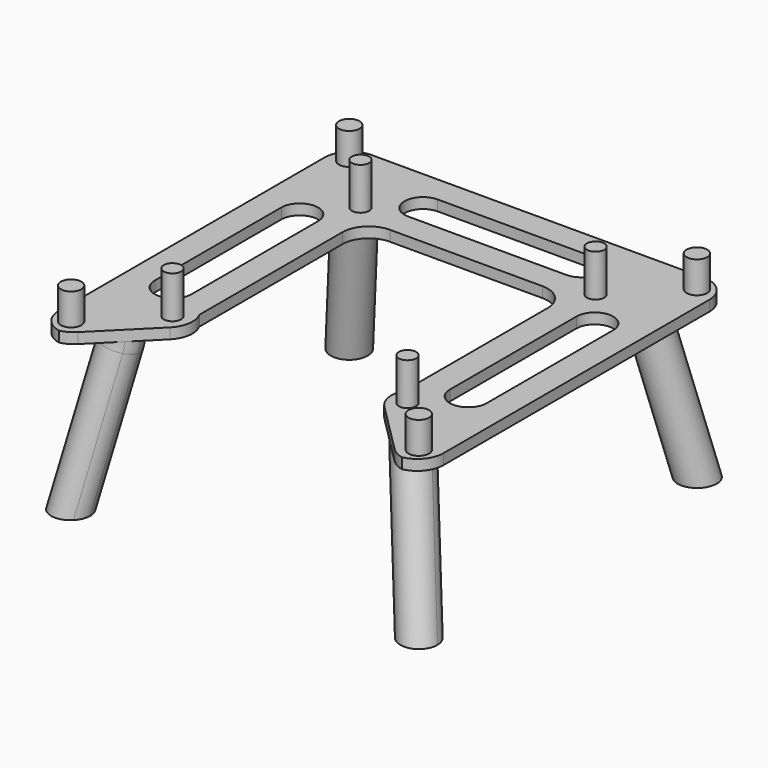
from build123d import *

# Parameters (mm, degrees)
F0_R           = 1.95
F0_R_2         = 1.65
F0_R_3         = 3.5355339059
F1_DEPTH       = 2
F2_T1_DEPTH    = 43.5812984693
F2_T3_DEPTH    = 12.3553390593
F2_T5_DEPTH    = 27
F2_T7_DEPTH    = 2
F3_ANGLE       = 15
F4_DEPTH       = 30
F5_ANGLE       = 15
F6_ANGLE       = 15
F7_ANGLE       = 15
F8_DEPTH       = 30
F9_DEPTH       = 30
F10_DEPTH      = 30
F11_W          = 91.7069762945
F11_H          = 4.37906757
F12_DEPTH      = 40
F12_DEPTH_BACK = 40
F13_DEPTH      = 10
F14_DEPTH      = 8


# Not quite as in the source:
# - a fillet or chamfer that OpenCascade refuses, or shapes differently, is made with other operations: its cross-section is extruded or revolved along the edge and cut away or added


with BuildPart() as f1:
    # F0 (on Top) → F1 (new body)
    with BuildSketch(Plane.XY):
        Polygon((-19.4715728753, 19.4715728753), (19.4715728753, 19.4715728753), (19.4715728753, -19.4715728753), (14.4715728753, -19.4715728753), (25.1386562498, -30.1386562498), (31.5128463018, -36.5128463018), (36.5128463018, -36.5128463018), (36.5128463018, 36.5128463018), (-36.5128463018, 36.5128463018), (-36.5128463018, -36.5128463018), (-31.5128463018, -36.5128463018), (-25.138656198, -30.138656198), (-14.4715728753, -19.4715728753), (-19.4715728753, -19.4715728753), align=None)
        with Locations((-32.9773123959, -32.9773123959)):
            Circle(F0_R, mode=Mode.SUBTRACT)
        with BuildLine():
            ThreePointArc((-24.103122292, -27.638656198), (-24.3722487858, -28.9916464483), (-25.138656198, -30.138656198))
            ThreePointArc((-25.138656198, -30.138656198), (-30.9050636101, -26.2856659476), (-24.103122292, -27.638656198))
        make_face(mode=Mode.SUBTRACT)
        with Locations((-22.3, -22.3)):
            Circle(F0_R_2, mode=Mode.SUBTRACT)
        with Locations((32.9773123959, -32.9773123959)):
            Circle(F0_R, mode=Mode.SUBTRACT)
        with BuildLine():
            ThreePointArc((31.1741901039, -27.638656198), (28.9916464822, -30.9050635961), (25.1386562498, -30.1386562498))
            ThreePointArc((25.1386562498, -30.1386562498), (26.2856659138, -24.3722487998), (31.1741901039, -27.638656198))
        make_face(mode=Mode.SUBTRACT)
        with Locations((22.3, -22.3)):
            Circle(F0_R_2, mode=Mode.SUBTRACT)
        with BuildLine():
            Line((-31.4922095886, -15), (-31.4922095886, 15))
            ThreePointArc((-31.4922095886, 15), (-27.9922095886, 18.5), (-24.4922095886, 15))
            Line((-24.4922095886, 15), (-24.4922095886, -15))
            ThreePointArc((-24.4922095886, -15), (-27.9922095886, -18.5), (-31.4922095886, -15))
        make_face(mode=Mode.SUBTRACT)
        with Locations((-22.3, 22.3)):
            Circle(F0_R_2, mode=Mode.SUBTRACT)
        with Locations((-27.638656198, 27.638656198)):
            Circle(F0_R_3, mode=Mode.SUBTRACT)
        with Locations((-32.9773123959, 32.9773123959)):
            Circle(F0_R, mode=Mode.SUBTRACT)
        with BuildLine():
            Line((31.4922095886, 15), (31.4922095886, -15))
            ThreePointArc((31.4922095886, -15), (27.9922095886, -18.5), (24.4922095886, -15))
            Line((24.4922095886, -15), (24.4922095886, 15))
            ThreePointArc((24.4922095886, 15), (27.9922095886, 18.5), (31.4922095886, 15))
        make_face(mode=Mode.SUBTRACT)
        with BuildLine():
            Line((-15, 31.4922095886), (15, 31.4922095886))
            ThreePointArc((15, 31.4922095886), (18.5, 27.9922095886), (15, 24.4922095886))
            Line((15, 24.4922095886), (-15, 24.4922095886))
            ThreePointArc((-15, 24.4922095886), (-18.5, 27.9922095886), (-15, 31.4922095886))
        make_face(mode=Mode.SUBTRACT)
        with Locations((22.3, 22.3)):
            Circle(F0_R_2, mode=Mode.SUBTRACT)
        with Locations((27.638656198, 27.638656198)):
            Circle(F0_R_3, mode=Mode.SUBTRACT)
        with Locations((32.9773123959, 32.9773123959)):
            Circle(F0_R, mode=Mode.SUBTRACT)
        with BuildLine():
            ThreePointArc((-24.103122292, -27.638656198), (-30.9050636101, -26.2856659476), (-25.138656198, -30.138656198))
            ThreePointArc((-25.138656198, -30.138656198), (-24.3722487858, -28.9916464483), (-24.103122292, -27.638656198))
        make_face()
        with Locations((-27.638656198, 27.638656198)):
            Circle(F0_R_3)
        with BuildLine():
            ThreePointArc((31.1741901039, -27.638656198), (26.2856659138, -24.3722487998), (25.1386562498, -30.1386562498))
            ThreePointArc((25.1386562498, -30.1386562498), (28.9916464822, -30.9050635961), (31.1741901039, -27.638656198))
        make_face()
        with Locations((27.638656198, 27.638656198)):
            Circle(F0_R_3)
    extrude(amount=F1_DEPTH)

    # F2: fillet of radius 5 on 10 edges, made by hand

    # F2_s2 → F2_t1 (cut)
    with BuildSketch(Plane.XY.offset(-20.7906492346)):
        with BuildLine():
            ThreePointArc((-20.3520564989, -25.3520564989), (-18.9427128058, -22.5569181158), (-19.4715728753, -19.4715728753))
            Line((-19.4715728753, -19.4715728753), (-19.3832525247, -19.4246738809))
            ThreePointArc((-19.3832525247, -19.4246738809), (-16.9715728753, -19.3715728753), (-14.4715728753, -19.3715728753))
            Line((-14.4715728753, -19.3715728753), (-14.4008621971, -19.5422835534))
            Line((-14.4008621971, -19.5422835534), (-20.2813458208, -25.422767177))
            Line((-20.2813458208, -25.422767177), (-20.3520564989, -25.3520564989))
        make_face()
        with BuildLine():
            ThreePointArc((20.3520564989, -25.3520564989), (18.9427128058, -22.5569181158), (19.4715728753, -19.4715728753))
            Line((19.4715728753, -19.4715728753), (19.3832525247, -19.4246738809))
            ThreePointArc((19.3832525247, -19.4246738809), (16.9715728753, -19.3715728753), (14.4715728753, -19.3715728753))
            Line((14.4715728753, -19.3715728753), (14.4008621971, -19.5422835534))
            Line((14.4008621971, -19.5422835534), (20.2813458208, -25.422767177))
            Line((20.2813458208, -25.422767177), (20.3520564989, -25.3520564989))
        make_face()
    extrude(amount=F2_T1_DEPTH, mode=Mode.SUBTRACT)

    # F2_s4 → F2_t3 (cut)
    with BuildSketch(Plane.XY.offset(-5.1776695297)):
        with BuildLine():
            ThreePointArc((-33.5839141137, -36.5128463018), (-31.6704969519, -36.1322439644), (-30.0483802078, -35.0483802078))
            Line((-30.0483802078, -35.0483802078), (-29.9776695297, -35.1190908859))
            Line((-29.9776695297, -35.1190908859), (-31.4714249456, -36.6128463018))
            Line((-31.4714249456, -36.6128463018), (-33.5839141137, -36.6128463018))
            Line((-33.5839141137, -36.6128463018), (-33.5839141137, -36.5128463018))
        make_face()
        with BuildLine():
            ThreePointArc((30.0483802078, -35.0483802078), (31.6704969519, -36.1322439644), (33.5839141137, -36.5128463018))
            Line((33.5839141137, -36.5128463018), (33.5839141137, -36.6128463018))
            Line((33.5839141137, -36.6128463018), (31.4714249456, -36.6128463018))
            Line((31.4714249456, -36.6128463018), (29.9776695297, -35.1190908859))
            Line((29.9776695297, -35.1190908859), (30.0483802078, -35.0483802078))
        make_face()
    extrude(amount=F2_T3_DEPTH, mode=Mode.SUBTRACT)

    # F2_s6 → F2_t5 (cut)
    with BuildSketch(Plane.XY.offset(-12.5)):
        with BuildLine():
            ThreePointArc((-36.5128463018, -31.5128463018), (-35.0483802078, -35.0483802078), (-31.5128463018, -36.5128463018))
            Line((-31.5128463018, -36.5128463018), (-31.5128463018, -36.6128463018))
            Line((-31.5128463018, -36.6128463018), (-36.6128463018, -36.6128463018))
            Line((-36.6128463018, -36.6128463018), (-36.6128463018, -31.5128463018))
            Line((-36.6128463018, -31.5128463018), (-36.5128463018, -31.5128463018))
        make_face()
        with BuildLine():
            ThreePointArc((31.5128463018, -36.5128463018), (35.0483802078, -35.0483802078), (36.5128463018, -31.5128463018))
            Line((36.5128463018, -31.5128463018), (36.6128463018, -31.5128463018))
            Line((36.6128463018, -31.5128463018), (36.6128463018, -36.6128463018))
            Line((36.6128463018, -36.6128463018), (31.5128463018, -36.6128463018))
            Line((31.5128463018, -36.6128463018), (31.5128463018, -36.5128463018))
        make_face()
        with BuildLine():
            ThreePointArc((36.5128463018, 31.5128463018), (35.0483802078, 35.0483802078), (31.5128463018, 36.5128463018))
            Line((31.5128463018, 36.5128463018), (31.5128463018, 36.6128463018))
            Line((31.5128463018, 36.6128463018), (36.6128463018, 36.6128463018))
            Line((36.6128463018, 36.6128463018), (36.6128463018, 31.5128463018))
            Line((36.6128463018, 31.5128463018), (36.5128463018, 31.5128463018))
        make_face()
        with BuildLine():
            ThreePointArc((-31.5128463018, 36.5128463018), (-35.0483802078, 35.0483802078), (-36.5128463018, 31.5128463018))
            Line((-36.5128463018, 31.5128463018), (-36.6128463018, 31.5128463018))
            Line((-36.6128463018, 31.5128463018), (-36.6128463018, 36.6128463018))
            Line((-36.6128463018, 36.6128463018), (-31.5128463018, 36.6128463018))
            Line((-31.5128463018, 36.6128463018), (-31.5128463018, 36.5128463018))
        make_face()
    extrude(amount=F2_T5_DEPTH, mode=Mode.SUBTRACT)

    # F2_s8 → F2_t7 (join)
    with BuildSketch(Plane.XY):
        with BuildLine():
            ThreePointArc((-14.4715728753, 19.4715728753), (-18.0071067812, 18.0071067812), (-19.4715728753, 14.4715728753))
            Line((-19.4715728753, 14.4715728753), (-19.5715728753, 14.4715728753))
            Line((-19.5715728753, 14.4715728753), (-19.5715728753, 19.5715728753))
            Line((-19.5715728753, 19.5715728753), (-14.4715728753, 19.5715728753))
            Line((-14.4715728753, 19.5715728753), (-14.4715728753, 19.4715728753))
        make_face()
        with BuildLine():
            ThreePointArc((19.4715728753, 14.4715728753), (18.0071067812, 18.0071067812), (14.4715728753, 19.4715728753))
            Line((14.4715728753, 19.4715728753), (14.4715728753, 19.5715728753))
            Line((14.4715728753, 19.5715728753), (19.5715728753, 19.5715728753))
            Line((19.5715728753, 19.5715728753), (19.5715728753, 14.4715728753))
            Line((19.5715728753, 14.4715728753), (19.4715728753, 14.4715728753))
        make_face()
    extrude(amount=F2_T7_DEPTH)

    # F0 (on Top) → F3 (revolve)
    with BuildSketch(Plane.XY):
        with BuildLine():
            ThreePointArc((-24.103122292, -27.638656198), (-30.9050636101, -26.2856659476), (-25.138656198, -30.138656198))
            ThreePointArc((-25.138656198, -30.138656198), (-24.3722487858, -28.9916464483), (-24.103122292, -27.638656198))
        make_face()
    revolve(axis=Axis((-36.4036751563, -29.5509496356, 0), (-0.7071067812, 0.7071067812, 0)), revolution_arc=F3_ANGLE)

    # F4 (add): a face of the model
    f4_faces = [f1.faces().sort_by_distance(p)[0] for p in [
        (-27.8205664966, -27.8205664966, -1.9540837905),
    ]]
    extrude(f4_faces, amount=F4_DEPTH)

    # F0 (on Top) → F5 (revolve)
    with BuildSketch(Plane.XY):
        with Locations((-27.638656198, 27.638656198)):
            Circle(F0_R_3)
    revolve(axis=Axis((-29.5509496356, 36.4036751563, 0), (0.7071067812, 0.7071067812, 0)), revolution_arc=F5_ANGLE)

    # F0 (on Top) → F6 (revolve)
    with BuildSketch(Plane.XY):
        with Locations((27.638656198, 27.638656198)):
            Circle(F0_R_3)
    revolve(axis=Axis((36.4036751563, 29.5509496356, 0), (0.7071067812, -0.7071067812, 0)), revolution_arc=F6_ANGLE)

    # F0 (on Top) → F7 (revolve)
    with BuildSketch(Plane.XY):
        with BuildLine():
            ThreePointArc((31.1741901039, -27.638656198), (26.2856659138, -24.3722487998), (25.1386562498, -30.1386562498))
            ThreePointArc((25.1386562498, -30.1386562498), (28.9916464822, -30.9050635961), (31.1741901039, -27.638656198))
        make_face()
    revolve(axis=Axis((29.5509496356, -36.4036751563, 0), (-0.7071067812, -0.7071067812, 0)), revolution_arc=F7_ANGLE)

    # F8 (add): a face of the model
    f8_faces = [f1.faces().sort_by_distance(p)[0] for p in [
        (-27.8205664966, 27.8205664966, -1.9540837905),
    ]]
    extrude(f8_faces, amount=F8_DEPTH)

    # F9 (add): a face of the model
    f9_faces = [f1.faces().sort_by_distance(p)[0] for p in [
        (27.8205664966, 27.8205664966, -1.9540837905),
    ]]
    extrude(f9_faces, amount=F9_DEPTH)

    # F10 (add): a face of the model
    f10_faces = [f1.faces().sort_by_distance(p)[0] for p in [
        (27.8205664966, -27.8205664966, -1.9540837905),
    ]]
    extrude(f10_faces, amount=F10_DEPTH)

    # F11 (on Right) → F12 (cut, two sides)
    with BuildSketch(Plane.YZ) as f12_sk:
        with Locations((0, -31.5507426858)):
            Rectangle(F11_W, F11_H)
    extrude(amount=-F12_DEPTH, mode=Mode.SUBTRACT)
    extrude(f12_sk.sketch, amount=F12_DEPTH_BACK, mode=Mode.SUBTRACT)


with BuildPart() as f13:
    # F0 (on Top) → F13 (new body)
    with BuildSketch(Plane.XY):
        with Locations((22.3, -22.3)):
            Circle(F0_R_2)
    extrude(amount=F13_DEPTH)


with BuildPart() as f13b:
    # F0 (on Top) → F13, piece 2 (new body)
    with BuildSketch(Plane.XY):
        with Locations((-22.3, -22.3)):
            Circle(F0_R_2)
    extrude(amount=F13_DEPTH)


with BuildPart() as f13c:
    # F0 (on Top) → F13, piece 3 (new body)
    with BuildSketch(Plane.XY):
        with Locations((-22.3, 22.3)):
            Circle(F0_R_2)
    extrude(amount=F13_DEPTH)


with BuildPart() as f13d:
    # F0 (on Top) → F13, piece 4 (new body)
    with BuildSketch(Plane.XY):
        with Locations((22.3, 22.3)):
            Circle(F0_R_2)
    extrude(amount=F13_DEPTH)


with BuildPart() as f14:
    # F0 (on Top) → F14 (new body)
    with BuildSketch(Plane.XY):
        with Locations((32.9773123959, -32.9773123959)):
            Circle(F0_R)
    extrude(amount=F14_DEPTH)


with BuildPart() as f14b:
    # F0 (on Top) → F14, piece 2 (new body)
    with BuildSketch(Plane.XY):
        with Locations((32.9773123959, 32.9773123959)):
            Circle(F0_R)
    extrude(amount=F14_DEPTH)


with BuildPart() as f14c:
    # F0 (on Top) → F14, piece 3 (new body)
    with BuildSketch(Plane.XY):
        with Locations((-32.9773123959, 32.9773123959)):
            Circle(F0_R)
    extrude(amount=F14_DEPTH)


with BuildPart() as f14d:
    # F0 (on Top) → F14, piece 4 (new body)
    with BuildSketch(Plane.XY):
        with Locations((-32.9773123959, -32.9773123959)):
            Circle(F0_R)
    extrude(amount=F14_DEPTH)


solid = Compound([f1.part, f13.part, f13b.part, f13c.part, f13d.part, f14.part, f14b.part, f14c.part, f14d.part])
